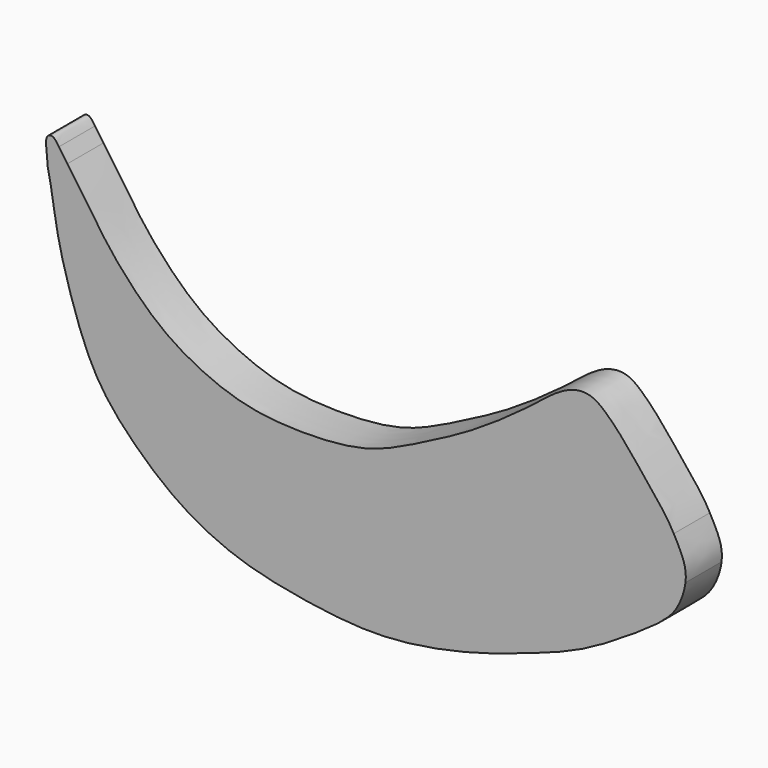
from build123d import *

# Parameters (mm, degrees)
F1_DEPTH = 1.5


with BuildPart() as f1:
    # F0 (on Front) → F1 (new body)
    with BuildSketch(Plane.XZ):
        with BuildLine():
            add(Edge.make_bspline(
                [(-15.5886812717, 11.4794949823), (-15.4143296847, 11.2382539811), (-15.0361844262, 10.7150345355), (-14.3520272629, 9.6369158456), (-13.3901809462, 8.4961422482), (-12.1013087962, 7.3193862365), (-10.0843733619, 6.363980171), (-8.321372324, 6.1358495153), (-6.5126508034, 6.1753650592), (-5.1529070228, 6.4692660827), (-3.5419333867, 7.2903643377), (-2.0612605045, 8.0556770571), (-0.2510856551, 9.3241557763), (0.5687606343, 10.0334130257), (1.2462094689, 10.3912597961), (1.8789769228, 10.3955484825), (2.442581301, 9.9073187544), (3.0325423811, 9.2674548808), (3.8016255024, 8.2778595229), (4.3631617457, 7.6096235524), (4.5653669513, 7.2100887828)],
                knots=[0, 0, 0, 0, 0.0212712459, 0.0461344856, 0.0730651165, 0.1023249612, 0.1350350284, 0.1647196312, 0.1940312263, 0.2201164738, 0.2492921901, 0.2785567502, 0.3112769334, 0.3344058624, 0.3531170279, 0.369878703, 0.3883554579, 0.4090860244, 0.4338064524, 0.4592890108, 0.4592890108, 0.4592890108, 0.4592890108], degree=3))
            add(Edge.make_bspline(
                [(-15.8734871656, 11.8816214435), (-15.8360353147, 11.825599868), (-15.7551088144, 11.7045476383), (-15.6468429454, 11.5581444589), (-15.5886812717, 11.4794949823)],
                knots=[0, 0, 0, 0, 0.4627884651, 1, 1, 1, 1], degree=3))
            add(Edge.make_bspline(
                [(-16.2409348995, 11.1616010599), (-16.2703143769, 11.4241276451), (-16.3163105059, 11.8351358634), (-16.2766238455, 12.0985623317), (-16.0542989155, 12.1625521871), (-15.9402444972, 11.985343612), (-15.8734871656, 11.8816214435)],
                knots=[0, 0, 0, 0, 0.3687463789, 0.5773045503, 0.7525916077, 1, 1, 1, 1], degree=3))
            add(Edge.make_bspline(
                [(4.0222675889, 4.4009554021), (3.6021214232, 4.0879163566), (2.711392987, 3.5070019245), (1.3858615233, 2.7255840104), (-0.2348494988, 2.1469154815), (-1.7808518748, 1.6221260795), (-3.4857384395, 1.214002475), (-5.5234793136, 0.976041948), (-7.8949454527, 1.2787065655), (-9.9769000961, 1.728705851), (-11.8276981969, 2.6487308245), (-13.3312194271, 3.9173596525), (-14.6651416452, 5.4067950099), (-15.4092058722, 7.3781913671), (-15.9673503273, 9.3212581102), (-16.1201270994, 10.6644633604), (-16.2409348995, 11.1616010599)],
                knots=[0.5275853115, 0.5275853115, 0.5275853115, 0.5275853115, 0.5553491604, 0.5827901242, 0.6116623363, 0.6399103515, 0.6689776706, 0.7006114359, 0.7347748549, 0.7670917923, 0.7985471692, 0.8294539301, 0.8604544038, 0.8923225225, 0.9241583255, 0.9538621091, 0.9538621091, 0.9538621091, 0.9538621091], degree=3))
            add(Edge.make_bspline(
                [(4.0222675889, 4.4009554021), (4.2126258121, 4.5540553088), (4.6001057654, 4.8656948253), (4.8703118565, 5.4594945664), (4.9442704879, 5.8067642972), (4.9558935946, 5.904401992)],
                knots=[0, 0, 0, 0, 0.2397665322, 0.488052069, 0.5846377064, 0.5846377064, 0.5846377064, 0.5846377064], degree=3))
            add(Edge.make_bspline(
                [(4.5653669513, 7.2100887828), (4.7618312787, 6.8218973434), (4.8919183573, 6.3322829413), (4.9512804987, 5.9393771693), (4.9558935946, 5.904401992)],
                knots=[0.4592890108, 0.4592890108, 0.4592890108, 0.4592890108, 0.4840480851, 0.4865206827, 0.4865206827, 0.4865206827, 0.4865206827], degree=3))
        make_face()
        with BuildLine():
            add(Edge.make_bspline(
                [(4.9558935946, 5.904401992), (4.9731158076, 6.0490739131), (4.9651784758, 6.4713839037), (4.7236661883, 6.9176099233), (4.5653669513, 7.2100887828)],
                knots=[0.5846377064, 0.5846377064, 0.5846377064, 0.5846377064, 0.7277507707, 1, 1, 1, 1], degree=3))
            add(Edge.make_bspline(
                [(4.5653669513, 7.2100887828), (4.7618312787, 6.8218973434), (4.8919183573, 6.3322829413), (4.9512804987, 5.9393771693), (4.9558935946, 5.904401992)],
                knots=[0.4592890108, 0.4592890108, 0.4592890108, 0.4592890108, 0.4840480851, 0.4865206827, 0.4865206827, 0.4865206827, 0.4865206827], degree=3))
        make_face()
    extrude(amount=F1_DEPTH)


solid = f1.part
